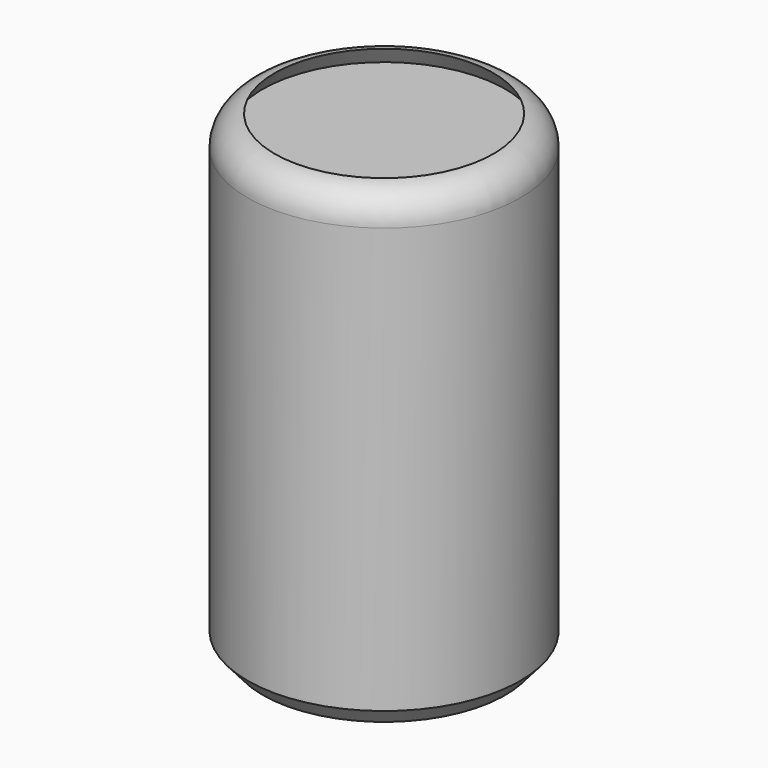
from build123d import *


# Not quite as in the source:
# - a fillet or chamfer that OpenCascade refuses, or shapes differently, is made with other operations: its cross-section is extruded or revolved along the edge and cut away or added


with BuildPart() as f1:
    # F0 (on Right) → F1 (revolve)
    with BuildSketch(Plane.YZ):
        Polygon((-20.1236736029, 0), (0, 0), (0, 75.3775425255), (-20.1236736029, 75.3775425255), (-18.1435449049, 78.3563926816), (-22.6185184726, 78.3563926816), (-22.6185184726, 2.8913898758), align=None)
    revolve(axis=Axis((0, 0, 37.6887712628), (0, 0, -1)))

    # F2: fillet of radius 5 on 1 edges, made by hand

    # F2_s1 → F2_t2 (revolve, cut)
    with BuildSketch(Plane.YZ):
        with BuildLine():
            ThreePointArc((-22.6185184726, 73.3840343633), (-21.3350445495, 76.7287965251), (-18.1435449049, 78.3563926816))
            Line((-18.1435449049, 78.3563926816), (-22.6185184726, 78.3563926816))
            Line((-22.6185184726, 78.3563926816), (-22.6185184726, 73.3840343633))
        make_face()
    revolve(axis=Axis((0, 0, 78.3563926816), (0, 0, -1)), mode=Mode.SUBTRACT)


solid = f1.part
